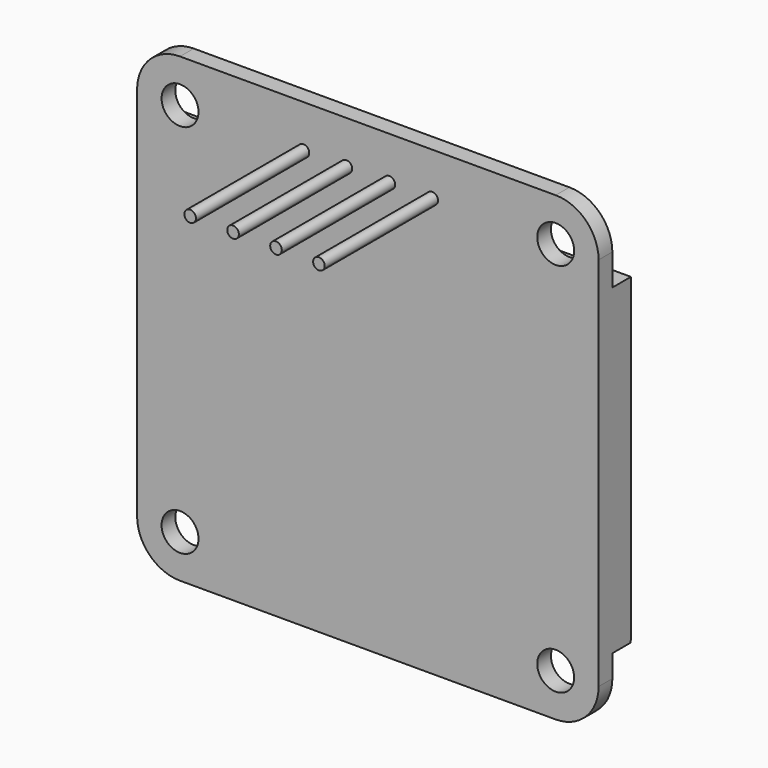
from build123d import *

# Parameters (mm, degrees)
F0_R        = 1.0922
F1_DEPTH    = 1.016
F2_R        = 0.3429
F3_DEPTH    = 8.382
F4_W        = 27.305
F4_H        = 19.05
F5_DEPTH    = 1.3716
F6_W        = 12.7
F6_H        = 3.8608
F7_DEPTH    = 1.3716
F8_T1_DEPTH = 34.2391400943


# Not quite as in the source:
# - a fillet or chamfer that OpenCascade refuses, or shapes differently, is made with other operations: its cross-section is extruded or revolved along the edge and cut away or added


with BuildPart() as f1:
    # F0 (on Front) → F1 (new body)
    with BuildSketch(Plane.XZ):
        with BuildLine():
            Line((11.1125, 13.6525), (-11.1125, 13.6525))
            ThreePointArc((-11.1125, 13.6525), (-12.9085512242, 12.9085512242), (-13.6525, 11.1125))
            Line((-13.6525, 11.1125), (-13.6525, -11.1125))
            ThreePointArc((-13.6525, -11.1125), (-12.9085512242, -12.9085512242), (-11.1125, -13.6525))
            Line((-11.1125, -13.6525), (11.1125, -13.6525))
            ThreePointArc((11.1125, -13.6525), (12.9085512242, -12.9085512242), (13.6525, -11.1125))
            Line((13.6525, -11.1125), (13.6525, 11.1125))
            ThreePointArc((13.6525, 11.1125), (12.9085512242, 12.9085512242), (11.1125, 13.6525))
        make_face()
        with Locations((-11.1125, -11.1125)):
            Circle(F0_R, mode=Mode.SUBTRACT)
        with Locations((11.1125, -11.1125)):
            Circle(F0_R, mode=Mode.SUBTRACT)
        with Locations((-11.1125, 11.1125)):
            Circle(F0_R, mode=Mode.SUBTRACT)
        with Locations((11.1125, 11.1125)):
            Circle(F0_R, mode=Mode.SUBTRACT)
    extrude(amount=F1_DEPTH)

    # F2 (on face) → F3 (join)
    with BuildSketch(Plane.XZ.offset(1.016)):
        with Locations((-3.81, 11.1125)):
            Circle(F2_R)
        with Locations((-1.27, 11.1125)):
            Circle(F2_R)
        with Locations((3.81, 11.1125)):
            Circle(F2_R)
        with Locations((1.27, 11.1125)):
            Circle(F2_R)
    extrude(amount=F3_DEPTH)

    # F4 (on face) → F5 (join)
    with BuildSketch(Plane(origin=(0, 0, 0), x_dir=(-1, 0, 0), z_dir=(0, 1, 0))):
        with Locations((0, -0.2667)):
            Rectangle(F4_W, F4_H)
    extrude(amount=F5_DEPTH)

    # F6 (on face) → F7 (join, through all)
    with BuildSketch(Plane(origin=(0, 0, 0), x_dir=(-1, 0, 0), z_dir=(0, 1, 0))):
        with Locations((0.0635, -11.7221)):
            Rectangle(F6_W, F6_H)
    extrude(amount=F7_DEPTH)

    # F8: fillet of radius 5.08 on 1 edges, made by hand

    # F8_s2 → F8_t1 (cut)
    with BuildSketch(Plane.YZ.offset(-17.1830700471)):
        with BuildLine():
            ThreePointArc((1.3716, -9.3446719811), (0.7347853439, -11.8072933487), (-1.016, -13.6525))
            Line((-1.016, -13.6525), (1.3716, -13.6525))
            Line((1.3716, -13.6525), (1.3716, -9.3446719811))
        make_face()
    extrude(amount=F8_T1_DEPTH, mode=Mode.SUBTRACT)


solid = f1.part
